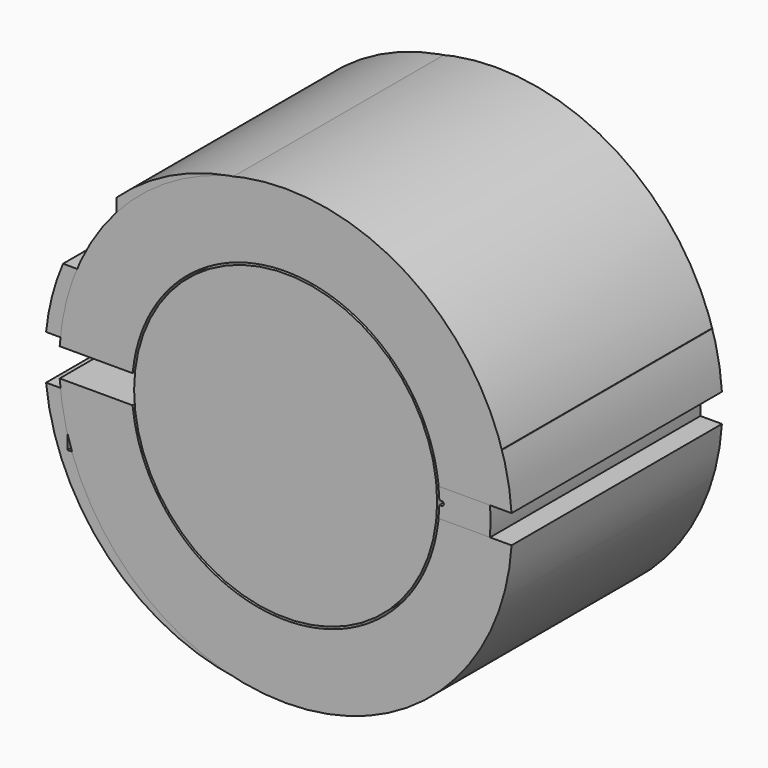
from build123d import *

# Parameters (mm, degrees)
F0_R      = 17
F1_DEPTH  = 29.5
F2_R      = 4.5
F3_DEPTH  = 13.7
F5_DEPTH  = 10.5
F7_DEPTH  = 29.5
F9_DEPTH  = 29.5
F10_R     = 1.5
F11_DEPTH = 21.59
F12_W     = 5.02
F12_H     = 2.7
F13_DEPTH = 29.5
F15_DEPTH = 29.5


# Not quite as in the source:
# - ends of sketch curves that miss each other by under 0.0002 mm in the source are joined


with BuildPart() as f1:
    # F0 (on Front) → F1 (new body)
    with BuildSketch(Plane.XZ):
        Circle(F0_R)
    extrude(amount=F1_DEPTH)

    # F2 (on face) → F3 (join)
    with BuildSketch(Plane(origin=(0, 0, 0), x_dir=(-1, 0, 0), z_dir=(0, 1, 0))):
        Circle(F2_R)
    extrude(amount=F3_DEPTH)

    # F4 (on face) → F5 (join)
    with BuildSketch(Plane(origin=(0, 13.7, 0), x_dir=(-1, 0, 0), z_dir=(0, 1, 0))):
        with BuildLine():
            Line((-4.5, 0), (-12.8, 0))
            ThreePointArc((-12.8, 0), (0, -12.8), (12.8, 0))
            Line((12.8, 0), (4.5, 0))
            Line((4.5, 0), (4.5, 4.5))
            Line((4.5, 4.5), (-4.5, 4.5))
            Line((-4.5, 4.5), (-4.5, 0))
        make_face()
    extrude(amount=-F5_DEPTH)


with BuildPart() as f7:
    # F6 (on face) → F7 (new body, through all)
    with BuildSketch(Plane(origin=(0, 0, 0), x_dir=(-1, 0, 0), z_dir=(0, 1, 0))):
        with BuildLine():
            Line((-24.2674679355, 7.5), (-24.2674679355, 2.5))
            Line((-24.2674679355, 2.5), (-17.0678791887, 2.5))
            ThreePointArc((-17.0678791887, 2.5), (0, 17.25), (17.0678791887, 2.5))
            Line((17.0678791887, 2.5), (24.2674679355, 2.5))
            Line((24.2674679355, 2.5), (24.2674679355, 7.5))
            Line((24.2674679355, 7.5), (20.9478519185, 7.5))
            ThreePointArc((20.9478519185, 7.5), (0, 22.25), (-20.9478519185, 7.5))
            Line((-20.9478519185, 7.5), (-24.2674679355, 7.5))
        make_face()
    extrude(amount=-F7_DEPTH)


with BuildPart() as f7b:
    # F6 (on face) → F7, piece 2 (new body, through all)
    with BuildSketch(Plane(origin=(0, 0, 0), x_dir=(-1, 0, 0), z_dir=(0, 1, 0))):
        with BuildLine():
            Line((24.2674679355, -2.5), (17.0678791887, -2.5))
            ThreePointArc((17.0678791887, -2.5), (0, -17.25), (-17.0678791887, -2.5))
            Line((-17.0678791887, -2.5), (-24.2674679355, -2.5))
            Line((-24.2674679355, -2.5), (-24.2674679355, -7.5))
            Line((-24.2674679355, -7.5), (-20.9478519185, -7.5))
            ThreePointArc((-20.9478519185, -7.5), (0, -22.25), (20.9478519185, -7.5))
            Line((20.9478519185, -7.5), (24.2674679355, -7.5))
            Line((24.2674679355, -7.5), (24.2674679355, -2.5))
        make_face()
    extrude(amount=-F7_DEPTH)


with BuildPart() as f9:
    # F8 (on face) → F9 (new body, through all)
    with BuildSketch(Plane.XZ.offset(29.5)):
        with BuildLine():
            Line((-17.0678791887, -2.5), (-26.8746859277, -2.5))
            ThreePointArc((-26.8746859277, -2.5), (21.377848053, -8.858680512), (-18.9712825582, 18.3568942997))
            Line((-18.9712825582, 18.3568942997), (-18.9712825582, 9.8650989672))
            Line((-18.9712825582, 9.8650989672), (-24.9712825582, 9.8650989672))
            ThreePointArc((-24.9712825582, 9.8650989672), (-26.2047587426, 6.2553700301), (-26.8746859277, 2.5))
            Line((-26.8746859277, 2.5), (-17.0678791887, 2.5))
            ThreePointArc((-17.0678791887, 2.5), (1.1286065944, 17.2130400323), (17.2481883107, 0.25))
            Line((17.2481883107, 0.25), (17.4941883107, 0.25))
            ThreePointArc((17.4941883107, 0.25), (17.6709438016, 0.1784102421), (17.7480624201, 0.0039960349))
            Line((17.7480624201, 0.0039960349), (17.7481883107, 0))
            Line((17.7481883107, 0), (17.7481883107, -0.004))
            ThreePointArc((17.7481883107, -0.004), (17.6709438016, -0.1784102421), (17.4941883107, -0.25))
            Line((17.4941883107, -0.25), (17.2481883107, -0.25))
            ThreePointArc((17.2481883107, -0.25), (1.1286065944, -17.2130400323), (-17.0678791887, -2.5))
        make_face()
    extrude(amount=-F9_DEPTH)

    # F10 (on face) → F11 (cut)
    with BuildSketch(Plane.XY.offset(9.8650989672)):
        with Locations((-21.9712825582, -7.375)):
            Circle(F10_R)
        with Locations((-21.9712825582, -22.125)):
            Circle(F10_R)
    extrude(amount=-F11_DEPTH, mode=Mode.SUBTRACT)

    # F12 (on face) → F13 (cut, through all)
    with BuildSketch(Plane(origin=(0, 0, 0), x_dir=(-1, 0, 0), z_dir=(0, 1, 0))):
        with Locations((21.9712825582, -7.025)):
            Rectangle(F12_W, F12_H)
    extrude(amount=-F13_DEPTH, mode=Mode.SUBTRACT)


with BuildPart() as f15:
    # F14 (on face) → F15 (new body, through all)
    with BuildSketch(Plane.XZ.offset(29.5)):
        with BuildLine():
            Line((-25.3503420835, 1.5875), (-17.1767966673, 1.5875))
            ThreePointArc((-17.1767966673, 1.5875), (0, 17.25), (17.1767966673, 1.5875))
            Line((17.1767966673, 1.5875), (25.3503420835, 1.5875))
            ThreePointArc((25.3503420835, 1.5875), (0, 25.4), (-25.3503420835, 1.5875))
        make_face()
    extrude(amount=-F15_DEPTH)


with BuildPart() as f15b:
    # F14 (on face) → F15, piece 2 (new body, through all)
    with BuildSketch(Plane.XZ.offset(29.5)):
        with BuildLine():
            ThreePointArc((17.1767966673, -1.5875), (0, -17.25), (-17.1767966673, -1.5875))
            Line((-17.1767966673, -1.5875), (-25.3503420835, -1.5875))
            ThreePointArc((-25.3503420835, -1.5875), (0, -25.4), (25.3503420835, -1.5875))
            Line((25.3503420835, -1.5875), (17.1767966673, -1.5875))
        make_face()
    extrude(amount=-F15_DEPTH)


solid = Compound([f1.part, f7.part, f7b.part, f9.part, f15.part, f15b.part])
